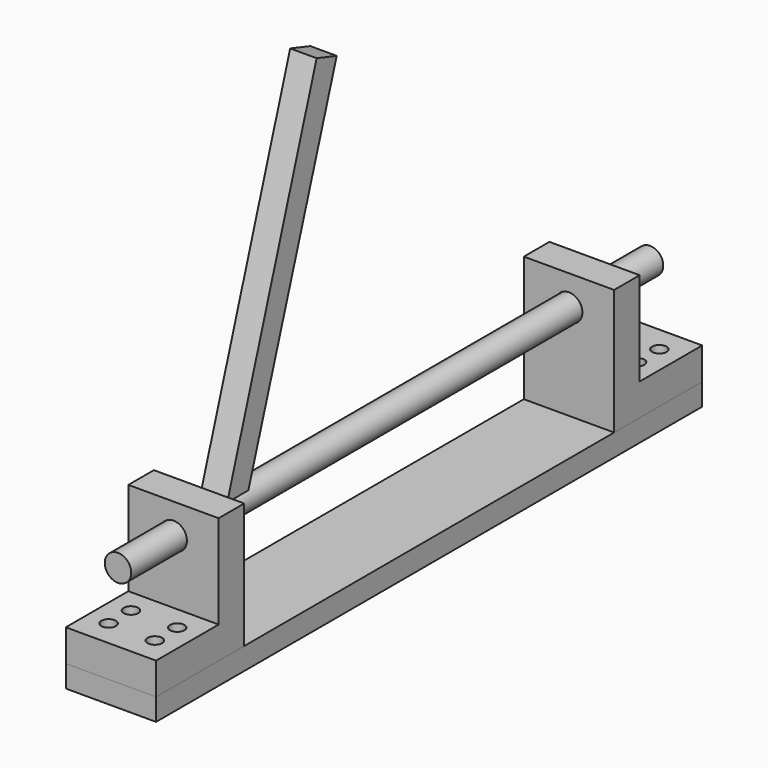
from build123d import *

# Parameters (mm, degrees)
F0_W           = 310
F0_H           = 10
F1_DEPTH       = 20.5
F1_DEPTH_BACK  = 20.5
F3_DEPTH       = 20.5
F3_DEPTH_BACK  = 20.5
F5_D           = 6.6
F5_2_D         = 6.6
F6_R           = 6.1
F7_DEPTH       = 25
F9_R           = 6
F10_DEPTH      = 151
F10_DEPTH_BACK = 151
F12_DEPTH      = 6
F12_DEPTH_BACK = 6


# Not quite as in the source:
# - a feature of the source that left no trace in its solid (it failed there, or was rolled back) is left out


with BuildPart() as f1:
    # F0 (on Right) → F1 (new body, two sides)
    with BuildSketch(Plane.YZ) as f1_sk:
        Rectangle(F0_W, F0_H)
    extrude(amount=F1_DEPTH)
    extrude(f1_sk.sketch, amount=-F1_DEPTH_BACK)

    # F5 (through all)
    with Locations(Plane.XY.offset(19.5)):
        with Locations((10.5, -143.2), (-10.5, -143.2), (-10.5, -130.5), (10.5, -130.5)):
            Hole(F5_D / 2)


with BuildPart() as f3:
    # F2 (on Right) → F3 (new body, two sides)
    with BuildSketch(Plane.YZ) as f3_sk:
        Polygon((-155, 19.5), (-155, 5), (-105, 5), (-105, 62), (-119.5, 62), (-119.5, 19.5), align=None)
    extrude(amount=F3_DEPTH)
    extrude(f3_sk.sketch, amount=-F3_DEPTH_BACK)

    # F5#2 (through all)
    with Locations(Plane.XY.offset(19.5)):
        with Locations((10.5, -143.2), (-10.5, -143.2), (-10.5, -130.5), (10.5, -130.5)):
            Hole(F5_2_D / 2)

    # F6 (on face) → F7 (cut)
    with BuildSketch(Plane(origin=(0, -105, 0), x_dir=(-1, 0, 0), z_dir=(0, 1, 0))):
        with Locations((0, 48.3)):
            Circle(F6_R)
    extrude(amount=-F7_DEPTH, mode=Mode.SUBTRACT)


with BuildPart() as f8_1:
    # F8: instance of F3
    add(f3.part.mirror(Plane.XZ))


with BuildPart() as f10:
    # F9 (on Front) → F10 (new body, two sides)
    with BuildSketch(Plane.XZ) as f10_sk:
        with Locations((0, 48.3)):
            Circle(F9_R)
    extrude(amount=F10_DEPTH)
    extrude(f10_sk.sketch, amount=-F10_DEPTH_BACK)

    # F11 (on Right) → F12 (join, two sides)
    with BuildSketch(Plane.YZ) as f12_sk:
        Polygon((-45.7456898382, 211.2), (-96.5, 54.2), (-84.5, 54.2), (-34.32750802, 207.5087774428), align=None)
    extrude(amount=F12_DEPTH)
    extrude(f12_sk.sketch, amount=-F12_DEPTH_BACK)


solid = Compound([f1.part, f3.part, f8_1.part, f10.part])
